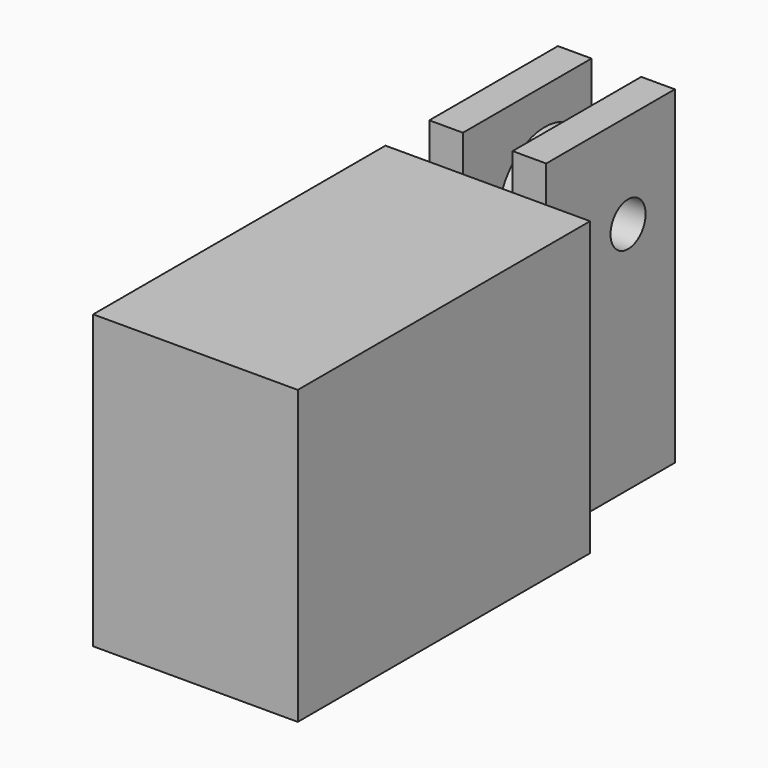
from build123d import *

# Parameters (mm, degrees)
F1_DEPTH = 11
F3_W     = 3
F3_H     = 20
F3_W_2   = 3.4
F3_H_2   = 10.2
F4_DEPTH = 25
F5_R     = 1.5
F6_DEPTH = 25
F5_R_2   = 2.5
F7_DEPTH = 8
F8_SIZE  = 1.49999
F9_SIZE  = 1.49999


# Not quite as in the source:
# - a fillet or chamfer is up to 0.001 mm smaller than in the source, because OpenCascade refuses the exact size


with BuildPart() as f1:
    # F0 (on Front) → F1 (new body)
    with BuildSketch(Plane.XZ):
        Polygon((-4, 0), (0, 0), (0, 9.8), (-1.7, 9.8), (-1.7, 22.5), (-4, 22.5), align=None)
    extrude(amount=F1_DEPTH)

    # F2: F1 across face


with BuildPart() as f1_1:
    add(f1.part)
    add(f1.part.mirror(Plane(origin=(0, -5.5, 4.9), x_dir=(0, 1, 0), z_dir=(1, 0, 0))))

    # F3 (on face) → F4 (join)
    with BuildSketch(Plane.XZ.offset(11)):
        with Locations((5.5, 10)):
            Rectangle(F3_W, F3_H)
        with Locations((0, 14.9)):
            Rectangle(F3_W_2, F3_H_2)
        Polygon((-4, 0), (0, 0), (4, 0), (4, 20), (1.7, 20), (1.7, 9.8), (-1.7, 9.8), (-1.7, 20), (-4, 20), align=None)
        with Locations((-5.5, 10)):
            Rectangle(F3_W, F3_H)
    extrude(amount=F4_DEPTH)

    # F5 (on face) → F6 (cut)
    with BuildSketch(Plane.YZ.offset(4)):
        with Locations((-4, 16)):
            Circle(F5_R)
    extrude(amount=-F6_DEPTH, mode=Mode.SUBTRACT)

    # F5 (on face) → F7 (join, through all)
    with BuildSketch(Plane.YZ.offset(4)):
        with Locations((-4, 16)):
            Circle(F5_R_2)
        with Locations((-4, 16)):
            Circle(F5_R, mode=Mode.SUBTRACT)
    extrude(amount=-F7_DEPTH)

    # F8 (size 1.5 in the source; OpenCascade refuses exactly that, so slightly less here)
    f8_edges = [f1_1.edges().sort_by_distance(p)[0] for p in [
        (-1.7, -6.5, 16),
    ]]
    chamfer(f8_edges, length=F8_SIZE)

    # F9 (size 1.5 in the source; OpenCascade refuses exactly that, so slightly less here)
    f9_edges = [f1_1.edges().sort_by_distance(p)[0] for p in [
        (1.7, -6.5, 16),
    ]]
    chamfer(f9_edges, length=F9_SIZE)


solid = f1_1.part
